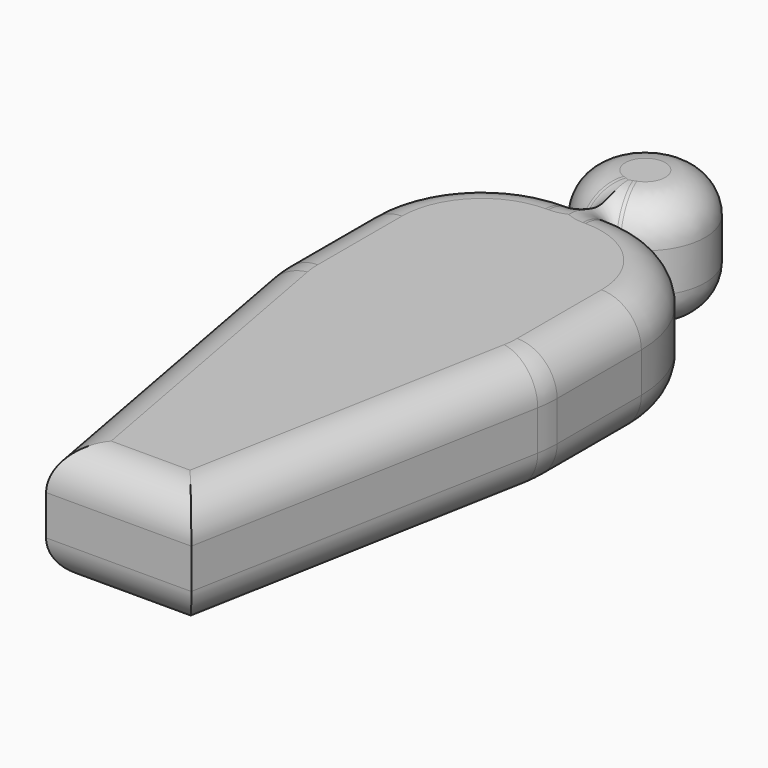
from build123d import *

# Parameters (mm, degrees)
F1_DEPTH     = 300
F2_R         = 300
F4_DEPTH     = 300
F5_T1_DEPTH  = 1146.4039437128
F5_T3_DEPTH  = 864.0548707486
F5_T5_DEPTH  = 1146.4039437128
F5_T7_DEPTH  = 263.9931695697
F5_T9_DEPTH  = 6.7787873377
F5_T11_DEPTH = 8.2506499138
F5_T13_DEPTH = 8.2506499138
F5_T15_DEPTH = 6.7787873377
F5_T18_ANGLE = 10.4750499308
F5_T20_ANGLE = 90
F5_T22_ANGLE = 160.5287793655
F5_T24_ANGLE = 321.057558731
F5_T26_ANGLE = 160.5287793655
F5_T28_ANGLE = 90
F5_T30_ANGLE = 10.4750499308
F5_T32_ANGLE = 10.4750499308
F5_T34_ANGLE = 90
F5_T36_ANGLE = 160.5287793655
F5_T38_ANGLE = 321.057558731
F5_T40_ANGLE = 160.5287793655
F5_T42_ANGLE = 90
F5_T44_ANGLE = 10.4750499308


# Not quite as in the source:
# - a fillet or chamfer that OpenCascade refuses, or shapes differently, is made with other operations: its cross-section is extruded or revolved along the edge and cut away or added


with BuildPart() as f1:
    # F0 (on Top) → F1 (new body)
    with BuildSketch(Plane.XY):
        Polygon((-182.0274353743, 0), (0, 0), (182.0274353743, 0), (350, 908.5065722466), (350, 1500), (-350, 1500), (-350, 908.5065722466), align=None)
    extrude(amount=F1_DEPTH)

    # F2
    f2_edges = [f1.edges().sort_by_distance(p)[0] for p in [
        (350, 1500, 150),
        (-350, 1500, 150),
        (-350, 908.506572, 150),
        (350, 908.506572, 150),
    ]]
    fillet(f2_edges, radius=F2_R)

    # F3 (on face) → F4 (join, through all)
    with BuildSketch(Plane.XY.offset(300)):
        with BuildLine():
            ThreePointArc((50, 1508.5786437627), (122.4744871392, 1563.3974596216), (150, 1650))
            ThreePointArc((150, 1650), (-86.6025403784, 1772.4744871392), (-50, 1508.5786437627))
            ThreePointArc((-50, 1508.5786437627), (0, 1500), (50, 1508.5786437627))
        make_face()
        with BuildLine():
            Line((42.2212126623, 1505.8284271247), (50, 1508.5786437627))
            ThreePointArc((50, 1508.5786437627), (25.3652965741, 1502.1602160117), (-4.764e-07, 1500))
            Line((-4.764e-07, 1500), (43.2212126623, 1500))
            ThreePointArc((43.2212126623, 1500), (40.2644169833, 1502.4926940638), (42.2212126623, 1505.8284271247))
        make_face()
        with BuildLine():
            ThreePointArc((-4.764e-07, 1500), (-25.3652970436, 1502.1602160923), (-50, 1508.5786437627))
            Line((-50, 1508.5786437627), (-42.2212126623, 1505.8284271247))
            ThreePointArc((-42.2212126623, 1505.8284271247), (-40.2644169834, 1502.4926940638), (-43.2212126623, 1500))
            Line((-43.2212126623, 1500), (-4.764e-07, 1500))
        make_face()
    extrude(amount=-F4_DEPTH)

    # F5: fillet of radius 100 on 32 edges, made by hand

    # F5_s2 → F5_t1 (cut)
    with BuildSketch(Plane(origin=(-168.9895340673, 914.0070146762, 0), x_dir=(0, 0, 1), z_dir=(0.1818073392, -0.9833341708, 0))):
        with BuildLine():
            ThreePointArc((100, 178.9937972219), (29.2893218813, 149.7044753406), (0, 78.9937972219))
            Line((0, 78.9937972219), (0, 178.9937972219))
            Line((0, 178.9937972219), (100, 178.9937972219))
        make_face()
        with BuildLine():
            ThreePointArc((200, 178.9937972219), (270.7106781187, 149.7044753406), (300, 78.9937972219))
            Line((300, 78.9937972219), (300, 178.9937972219))
            Line((300, 178.9937972219), (200, 178.9937972219))
        make_face()
    extrude(amount=F5_T1_DEPTH, mode=Mode.SUBTRACT)

    # F5_s4 → F5_t3 (cut)
    with BuildSketch(Plane.YZ.offset(-432.0274353743)):
        with BuildLine():
            ThreePointArc((100, 0), (29.2893218813, 29.2893218813), (0, 100))
            Line((0, 100), (0, 0))
            Line((0, 0), (100, 0))
        make_face()
        with BuildLine():
            ThreePointArc((0, 200), (29.2893218813, 270.7106781187), (100, 300))
            Line((100, 300), (0, 300))
            Line((0, 300), (0, 200))
        make_face()
    extrude(amount=F5_T3_DEPTH, mode=Mode.SUBTRACT)

    # F5_s6 → F5_t5 (cut)
    with BuildSketch(Plane(origin=(-39.4351165914, -213.2911566867, 0), x_dir=(0, 0, 1), z_dir=(0.1818073392, 0.9833341708, 0))):
        with BuildLine():
            ThreePointArc((0, 78.9937972219), (29.2893218813, 149.7044753406), (100, 178.9937972219))
            Line((100, 178.9937972219), (0, 178.9937972219))
            Line((0, 178.9937972219), (0, 78.9937972219))
        make_face()
        with BuildLine():
            ThreePointArc((300, 78.9937972219), (270.7106781187, 149.7044753406), (200, 178.9937972219))
            Line((200, 178.9937972219), (300, 178.9937972219))
            Line((300, 178.9937972219), (300, 78.9937972219))
        make_face()
    extrude(amount=F5_T5_DEPTH, mode=Mode.SUBTRACT)

    # F5_s8 → F5_t7 (cut)
    with BuildSketch(Plane.XZ.offset(-1200)):
        with BuildLine():
            ThreePointArc((250, 0), (320.7106781187, 29.2893218813), (350, 100))
            Line((350, 100), (350, 0))
            Line((350, 0), (250, 0))
        make_face()
        with BuildLine():
            ThreePointArc((-250, 0), (-320.7106781187, 29.2893218813), (-350, 100))
            Line((-350, 100), (-350, 0))
            Line((-350, 0), (-250, 0))
        make_face()
        with BuildLine():
            ThreePointArc((250, 300), (320.7106781187, 270.7106781187), (350, 200))
            Line((350, 200), (350, 300))
            Line((350, 300), (250, 300))
        make_face()
        with BuildLine():
            ThreePointArc((-250, 300), (-320.7106781187, 270.7106781187), (-350, 200))
            Line((-350, 200), (-350, 300))
            Line((-350, 300), (-250, 300))
        make_face()
    extrude(amount=F5_T7_DEPTH, mode=Mode.SUBTRACT)

    # F5_s10 → F5_t9 (cut)
    with BuildSketch(Plane.YZ.offset(43.2212126623)):
        with BuildLine():
            ThreePointArc((1400, 0), (1470.7106781187, 29.2893218813), (1500, 100))
            Line((1500, 100), (1500, 0))
            Line((1500, 0), (1400, 0))
        make_face()
        with BuildLine():
            ThreePointArc((1400, 300), (1470.7106781187, 270.7106781187), (1500, 200))
            Line((1500, 200), (1500, 300))
            Line((1500, 300), (1400, 300))
        make_face()
    extrude(amount=F5_T9_DEPTH, mode=Mode.SUBTRACT)

    # F5_s12 → F5_t11 (cut)
    with BuildSketch(Plane(origin=(510.7661855325, 180.5831166954, 0), x_dir=(0, 0, 1), z_dir=(0.9428090416, 0.3333333333, 0))):
        with BuildLine():
            ThreePointArc((0, -1505.6349186104), (29.2893218813, -1434.9242404917), (100, -1405.6349186104))
            Line((100, -1405.6349186104), (0, -1405.6349186104))
            Line((0, -1405.6349186104), (0, -1505.6349186104))
        make_face()
        with BuildLine():
            ThreePointArc((300, -1505.6349186104), (270.7106781187, -1434.9242404917), (200, -1405.6349186104))
            Line((200, -1405.6349186104), (300, -1405.6349186104))
            Line((300, -1405.6349186104), (300, -1505.6349186104))
        make_face()
    extrude(amount=F5_T11_DEPTH, mode=Mode.SUBTRACT)

    # F5_s14 → F5_t13 (cut)
    with BuildSketch(Plane(origin=(-518.5449728702, 183.3333333334, 0), x_dir=(0, 0, 1), z_dir=(0.9428090416, -0.3333333333, 0))):
        with BuildLine():
            ThreePointArc((0, -1505.6349186104), (29.2893218813, -1434.9242404917), (100, -1405.6349186104))
            Line((100, -1405.6349186104), (0, -1405.6349186104))
            Line((0, -1405.6349186104), (0, -1505.6349186104))
        make_face()
        with BuildLine():
            ThreePointArc((300, -1505.6349186104), (270.7106781187, -1434.9242404917), (200, -1405.6349186104))
            Line((200, -1405.6349186104), (300, -1405.6349186104))
            Line((300, -1405.6349186104), (300, -1505.6349186104))
        make_face()
    extrude(amount=F5_T13_DEPTH, mode=Mode.SUBTRACT)

    # F5_s16 → F5_t15 (cut)
    with BuildSketch(Plane.YZ.offset(-50)):
        with BuildLine():
            ThreePointArc((1400, 0), (1470.7106781187, 29.2893218813), (1500, 100))
            Line((1500, 100), (1500, 0))
            Line((1500, 0), (1400, 0))
        make_face()
        with BuildLine():
            ThreePointArc((1400, 300), (1470.7106781187, 270.7106781187), (1500, 200))
            Line((1500, 200), (1500, 300))
            Line((1500, 300), (1400, 300))
        make_face()
    extrude(amount=F5_T15_DEPTH, mode=Mode.SUBTRACT)

    # F5_s17 → F5_t18 (revolve, cut)
    with BuildSketch(Plane.XZ.offset(-936.0068304303)):
        with BuildLine():
            ThreePointArc((250, 0), (320.7106781187, 29.2893218813), (350, 100))
            Line((350, 100), (350, 0))
            Line((350, 0), (250, 0))
        make_face()
    revolve(axis=Axis((50, 936.0068304303, 0), (0, 0, -1)), revolution_arc=F5_T18_ANGLE, mode=Mode.SUBTRACT)

    # F5_s19 → F5_t20 (revolve, cut)
    with BuildSketch(Plane.YZ.offset(50)):
        with BuildLine():
            ThreePointArc((1400, 0), (1470.7106781187, 29.2893218813), (1500, 100))
            Line((1500, 100), (1500, 0))
            Line((1500, 0), (1400, 0))
        make_face()
    revolve(axis=Axis((50, 1200, 0), (0, 0, -1)), revolution_arc=F5_T20_ANGLE, mode=Mode.SUBTRACT)

    # F5_s21 → F5_t22 (revolve, cut)
    with BuildSketch(Plane.YZ.offset(43.2212126623)):
        with BuildLine():
            ThreePointArc((1400, 0), (1470.7106781187, 29.2893218813), (1500, 100))
            Line((1500, 100), (1500, 0))
            Line((1500, 0), (1400, 0))
        make_face()
    revolve(axis=Axis((43.2212126623, 1503, 0), (0, 0, -1)), revolution_arc=F5_T22_ANGLE, mode=Mode.SUBTRACT)

    # F5_s23 → F5_t24 (revolve, cut)
    with BuildSketch(Plane(origin=(518.5449728701, 183.3333333333, 0), x_dir=(0, 0, 1), z_dir=(-0.9428090416, -0.3333333333, 0))):
        with BuildLine():
            ThreePointArc((0, 1505.6349186104), (29.2893218813, 1434.9242404917), (100, 1405.6349186104))
            Line((100, 1405.6349186104), (0, 1405.6349186104))
            Line((0, 1405.6349186104), (0, 1505.6349186104))
        make_face()
    revolve(axis=Axis((0, 1650, 0), (0, 0, 1)), revolution_arc=F5_T24_ANGLE, mode=Mode.SUBTRACT)

    # F5_s25 → F5_t26 (revolve, cut)
    with BuildSketch(Plane(origin=(-510.7661855325, 180.5831166954, 0), x_dir=(0, 0, 1), z_dir=(-0.9428090416, 0.3333333333, 0))):
        with BuildLine():
            ThreePointArc((0, 1505.6349186104), (29.2893218813, 1434.9242404917), (100, 1405.6349186104))
            Line((100, 1405.6349186104), (0, 1405.6349186104))
            Line((0, 1405.6349186104), (0, 1505.6349186104))
        make_face()
    revolve(axis=Axis((-43.2212126623, 1503, 0), (0, 0, -1)), revolution_arc=F5_T26_ANGLE, mode=Mode.SUBTRACT)

    # F5_s27 → F5_t28 (revolve, cut)
    with BuildSketch(Plane.YZ.offset(-50)):
        with BuildLine():
            ThreePointArc((1400, 0), (1470.7106781187, 29.2893218813), (1500, 100))
            Line((1500, 100), (1500, 0))
            Line((1500, 0), (1400, 0))
        make_face()
    revolve(axis=Axis((-50, 1200, 0), (0, 0, 1)), revolution_arc=F5_T28_ANGLE, mode=Mode.SUBTRACT)

    # F5_s29 → F5_t30 (revolve, cut)
    with BuildSketch(Plane(origin=(-168.9895340673, 914.0070146762, 0), x_dir=(0, 0, 1), z_dir=(0.1818073392, -0.9833341708, 0))):
        with BuildLine():
            ThreePointArc((0, 78.9937972219), (29.2893218813, 149.7044753406), (100, 178.9937972219))
            Line((100, 178.9937972219), (0, 178.9937972219))
            Line((0, 178.9937972219), (0, 78.9937972219))
        make_face()
    revolve(axis=Axis((-50, 936.0068304303, 0), (0, 0, -1)), revolution_arc=F5_T30_ANGLE, mode=Mode.SUBTRACT)

    # F5_s31 → F5_t32 (revolve, cut)
    with BuildSketch(Plane.XZ.offset(-936.0068304303)):
        with BuildLine():
            ThreePointArc((250, 300), (320.7106781187, 270.7106781187), (350, 200))
            Line((350, 200), (350, 300))
            Line((350, 300), (250, 300))
        make_face()
    revolve(axis=Axis((50, 936.0068304303, 300), (0, 0, -1)), revolution_arc=F5_T32_ANGLE, mode=Mode.SUBTRACT)

    # F5_s33 → F5_t34 (revolve, cut)
    with BuildSketch(Plane.YZ.offset(50)):
        with BuildLine():
            ThreePointArc((1400, 300), (1470.7106781187, 270.7106781187), (1500, 200))
            Line((1500, 200), (1500, 300))
            Line((1500, 300), (1400, 300))
        make_face()
    revolve(axis=Axis((50, 1200, 300), (0, 0, -1)), revolution_arc=F5_T34_ANGLE, mode=Mode.SUBTRACT)

    # F5_s35 → F5_t36 (revolve, cut)
    with BuildSketch(Plane.YZ.offset(43.2212126623)):
        with BuildLine():
            ThreePointArc((1400, 300), (1470.7106781187, 270.7106781187), (1500, 200))
            Line((1500, 200), (1500, 300))
            Line((1500, 300), (1400, 300))
        make_face()
    revolve(axis=Axis((43.2212126623, 1503, 300), (0, 0, -1)), revolution_arc=F5_T36_ANGLE, mode=Mode.SUBTRACT)

    # F5_s37 → F5_t38 (revolve, cut)
    with BuildSketch(Plane(origin=(518.5449728701, 183.3333333333, 0), x_dir=(0, 0, 1), z_dir=(-0.9428090416, -0.3333333333, 0))):
        with BuildLine():
            ThreePointArc((300, 1505.6349186104), (270.7106781187, 1434.9242404917), (200, 1405.6349186104))
            Line((200, 1405.6349186104), (300, 1405.6349186104))
            Line((300, 1405.6349186104), (300, 1505.6349186104))
        make_face()
    revolve(axis=Axis((0, 1650, 300), (0, 0, 1)), revolution_arc=F5_T38_ANGLE, mode=Mode.SUBTRACT)

    # F5_s39 → F5_t40 (revolve, cut)
    with BuildSketch(Plane(origin=(-510.7661855325, 180.5831166954, 0), x_dir=(0, 0, 1), z_dir=(-0.9428090416, 0.3333333333, 0))):
        with BuildLine():
            ThreePointArc((300, 1505.6349186104), (270.7106781187, 1434.9242404917), (200, 1405.6349186104))
            Line((200, 1405.6349186104), (300, 1405.6349186104))
            Line((300, 1405.6349186104), (300, 1505.6349186104))
        make_face()
    revolve(axis=Axis((-43.2212126623, 1503, 300), (0, 0, -1)), revolution_arc=F5_T40_ANGLE, mode=Mode.SUBTRACT)

    # F5_s41 → F5_t42 (revolve, cut)
    with BuildSketch(Plane.YZ.offset(-50)):
        with BuildLine():
            ThreePointArc((1400, 300), (1470.7106781187, 270.7106781187), (1500, 200))
            Line((1500, 200), (1500, 300))
            Line((1500, 300), (1400, 300))
        make_face()
    revolve(axis=Axis((-50, 1200, 300), (0, 0, 1)), revolution_arc=F5_T42_ANGLE, mode=Mode.SUBTRACT)

    # F5_s43 → F5_t44 (revolve, cut)
    with BuildSketch(Plane(origin=(-168.9895340673, 914.0070146762, 0), x_dir=(0, 0, 1), z_dir=(0.1818073392, -0.9833341708, 0))):
        with BuildLine():
            ThreePointArc((200, 178.9937972219), (270.7106781187, 149.7044753406), (300, 78.9937972219))
            Line((300, 78.9937972219), (300, 178.9937972219))
            Line((300, 178.9937972219), (200, 178.9937972219))
        make_face()
    revolve(axis=Axis((-50, 936.0068304303, 300), (0, 0, -1)), revolution_arc=F5_T44_ANGLE, mode=Mode.SUBTRACT)


solid = f1.part
